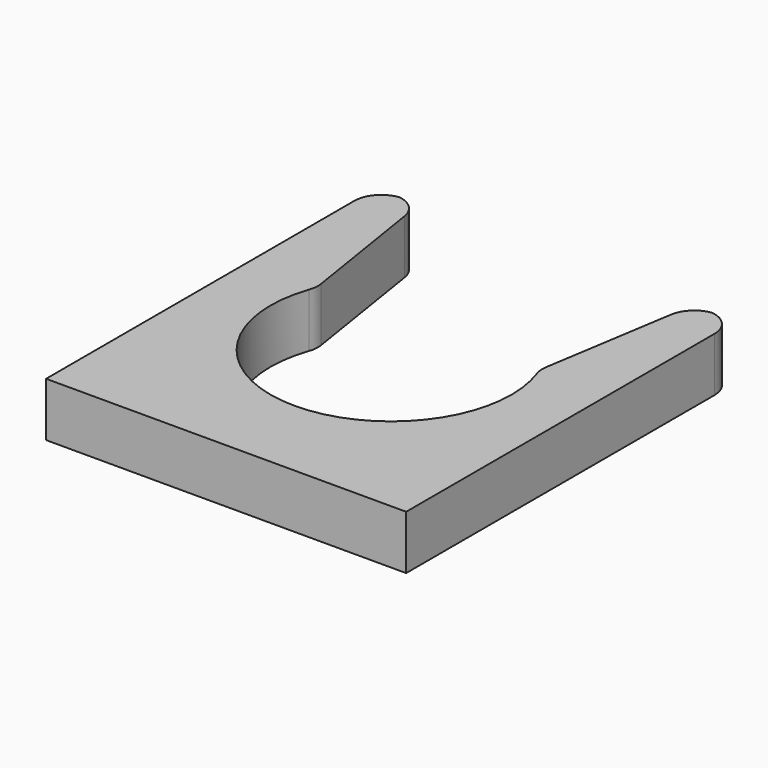
from build123d import *

# Parameters (mm, degrees)
F1_DEPTH    = 3.81
F2_T1_DEPTH = 11.945118529
F2_T3_DEPTH = 13.335
F2_T5_DEPTH = 6.3475490509


# Not quite as in the source:
# - a fillet or chamfer that OpenCascade refuses, or shapes differently, is made with other operations: its cross-section is extruded or revolved along the edge and cut away or added


with BuildPart() as f1:
    # F0 (on Top) → F1 (new body)
    with BuildSketch(Plane.XY):
        with BuildLine():
            ThreePointArc((7.8636785966, 3.2504830303), (0, -8.509), (-7.8636785966, 3.2504830303))
            Line((-7.8636785966, 3.2504830303), (-9.652, 14.5415))
            Line((-9.652, 14.5415), (-12.7, 14.5415))
            Line((-12.7, 14.5415), (-12.7, -14.5415))
            Line((-12.7, -14.5415), (12.7, -14.5415))
            Line((12.7, -14.5415), (12.7, 14.5415))
            Line((12.7, 14.5415), (9.652, 14.5415))
            Line((9.652, 14.5415), (7.8636785966, 3.2504830303))
        make_face()
    extrude(amount=F1_DEPTH)

    # F2: fillet of radius 1.905 on 6 edges, made by hand

    # F2_s2 → F2_t1 (cut)
    with BuildSketch(Plane.XY.offset(-4.0675592645)):
        with BuildLine():
            ThreePointArc((-9.397477417, 12.9345076559), (-10.0418251737, 14.0850733645), (-11.2790237058, 14.5415))
            Line((-11.2790237058, 14.5415), (-9.652, 14.5415))
            Line((-9.652, 14.5415), (-9.397477417, 12.9345076559))
        make_face()
        with BuildLine():
            ThreePointArc((11.2790237058, 14.5415), (10.0418251737, 14.0850733645), (9.397477417, 12.9345076559))
            Line((9.397477417, 12.9345076559), (9.652, 14.5415))
            Line((9.652, 14.5415), (11.2790237058, 14.5415))
        make_face()
    extrude(amount=F2_T1_DEPTH, mode=Mode.SUBTRACT)

    # F2_s4 → F2_t3 (cut)
    with BuildSketch(Plane.XY.offset(-4.7625)):
        with BuildLine():
            ThreePointArc((-10.795, 14.5415), (-12.1420384182, 13.9835384182), (-12.7, 12.6365))
            Line((-12.7, 12.6365), (-12.7, 14.5415))
            Line((-12.7, 14.5415), (-10.795, 14.5415))
        make_face()
        with BuildLine():
            ThreePointArc((12.7, 12.6365), (12.1420384182, 13.9835384182), (10.795, 14.5415))
            Line((10.795, 14.5415), (12.7, 14.5415))
            Line((12.7, 14.5415), (12.7, 12.6365))
        make_face()
    extrude(amount=F2_T3_DEPTH, mode=Mode.SUBTRACT)

    # F2_s6 → F2_t5 (cut)
    with BuildSketch(Plane.XY.offset(-1.2687745255)):
        with BuildLine():
            ThreePointArc((-8.0274308907, 2.821955757), (-7.9274098449, 3.2816022158), (-7.9430706222, 3.7517445525))
            Line((-7.9430706222, 3.7517445525), (-7.8636785966, 3.2504830303))
            ThreePointArc((-7.8636785966, 3.2504830303), (-7.9484431866, 3.0373231487), (-8.0274308907, 2.821955757))
        make_face()
        with BuildLine():
            ThreePointArc((8.0274308907, 2.821955757), (7.9274098449, 3.2816022158), (7.9430706222, 3.7517445525))
            Line((7.9430706222, 3.7517445525), (7.8636785966, 3.2504830303))
            ThreePointArc((7.8636785966, 3.2504830303), (7.9484431866, 3.0373231487), (8.0274308907, 2.821955757))
        make_face()
    extrude(amount=F2_T5_DEPTH, mode=Mode.SUBTRACT)


solid = f1.part
